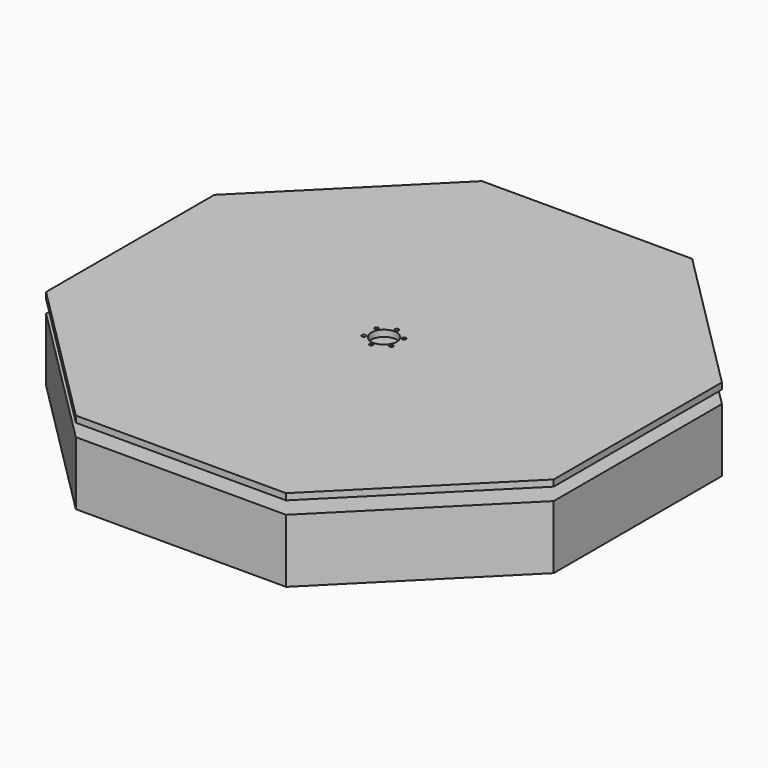
from build123d import *

# Parameters (mm, degrees)
F1_DEPTH = 50
F3_START = 10
F3_DEPTH = 5
F4_T     = -2.5
F5_R     = 10
F6_DEPTH = 65.001
F7_R     = 1.5
F8_DEPTH = 15
F9_SIZE  = 30
F10_SIZE = 5


with BuildPart() as f1:
    # F0 (on Top) → F1 (new body)
    with BuildSketch(Plane.XY):
        Polygon((200, -82.8427124746), (200, 82.8427124746), (82.8427124746, 200), (-82.8427124746, 200), (-200, 82.8427124746), (-200, -82.8427124746), (-82.8427124746, -200), (82.8427124746, -200), align=None)
    extrude(amount=-F1_DEPTH)

    # F4
    f4_openings = [f1.faces().sort_by_distance(p)[0] for p in [
        (0, 0, -50),
    ]]
    offset(amount=F4_T, openings=f4_openings)


with BuildPart() as f3:
    # F2 (on face) → F3 (new body)
    with BuildSketch(Plane.XY.offset(F3_START)):
        Polygon((82.8427124746, 200), (-82.8427124746, 200), (-200, 82.8427124746), (-200, -82.8427124746), (-82.8427124746, -200), (82.8427124746, -200), (200, -82.8427124746), (200, 82.8427124746), align=None)
    extrude(amount=F3_DEPTH)


with BuildPart() as f6_tool:
    # F5 (on face) → F6 (new body, through all)
    with BuildSketch(Plane.XY.offset(15)):
        Circle(F5_R)
    extrude(amount=-F6_DEPTH)


with BuildPart() as f1_1:
    add(f1.part)

    # F6: cut by f6_tool
    add(f6_tool.part, mode=Mode.SUBTRACT)

    # F9
    f9_edges = [f1_1.edges().sort_by_distance(p)[0] for p in [
        (-81.807179, -197.5, -26.25),
        (81.807179, -197.5, -26.25),
        (197.5, -81.807179, -26.25),
        (197.5, 81.807179, -26.25),
        (81.807179, 197.5, -26.25),
        (-81.807179, 197.5, -26.25),
        (-197.5, 81.807179, -26.25),
        (-197.5, -81.807179, -26.25),
    ]]
    chamfer(f9_edges, length=F9_SIZE)

    # F10
    f10_edges = [f1_1.edges().sort_by_distance(p)[0] for p in [
        (-139.653589, -139.653589, -2.5),
        (0, -197.5, -2.5),
        (139.653589, -139.653589, -2.5),
        (197.5, 0, -2.5),
        (139.653589, 139.653589, -2.5),
        (0, 197.5, -2.5),
        (-139.653589, 139.653589, -2.5),
        (-197.5, 0, -2.5),
    ]]
    chamfer(f10_edges, length=F10_SIZE)


with BuildPart() as f3_1:
    add(f3.part)

    # F6: cut by f6_tool
    add(f6_tool.part, mode=Mode.SUBTRACT)

    # F7 (on face) → F8 (cut)
    with BuildSketch(Plane.XY.offset(15)):
        with Locations((0, 12.5)):
            Circle(F7_R)
        with Locations((-10.8253174314, 6.2500002007)):
            Circle(F7_R)
        with Locations((-10.8253177791, -6.2499995985)):
            Circle(F7_R)
        with Locations((-6.954e-07, -12.5)):
            Circle(F7_R)
        with Locations((10.8253170837, -6.2500008029)):
            Circle(F7_R)
        with Locations((10.8253181268, 6.2499989963)):
            Circle(F7_R)
    extrude(amount=-F8_DEPTH, mode=Mode.SUBTRACT)


solid = Compound([f1_1.part, f3_1.part])
